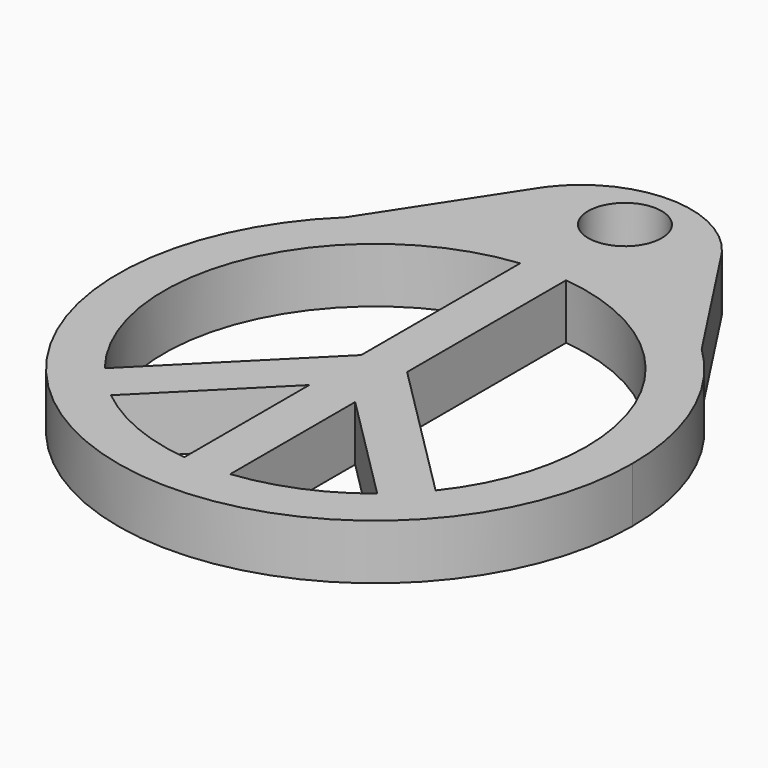
from build123d import *

# Parameters (mm, degrees)
F1_R     = 2
F2_DEPTH = 3


with BuildPart() as f2:
    # F1 (on Top) → F2 (new body)
    with BuildSketch(Plane.XY):
        with BuildLine():
            ThreePointArc((-9.7114153746, 10.0840672063), (-5.4790594428, -12.8833189676), (14, 0))
            ThreePointArc((14, 0), (12.8833189676, 5.4790594428), (9.7114153746, 10.0840672063))
            ThreePointArc((9.7114153746, 10.0840672063), (7.8963049332, 11.5606387541), (5.8606261419, 12.7142857143))
            ThreePointArc((5.8606261419, 12.7142857143), (0, 14), (-5.8606261419, 12.7142857143))
            ThreePointArc((-5.8606261419, 12.7142857143), (-7.8963049332, 11.5606387541), (-9.7114153746, 10.0840672063))
        make_face()
        with BuildLine():
            ThreePointArc((1.25, 11.4318633652), (8.5622718948, 7.6770762664), (11.5, 0))
            ThreePointArc((11.5, 0), (10.8590955773, -3.7855043577), (9.0078185666, -7.1490701963))
            ThreePointArc((9.0078185666, -7.1490701963), (8.1773610714, -8.0858373659), (7.25, -8.9267855357))
            ThreePointArc((7.25, -8.9267855357), (4.4307283524, -10.6121932826), (1.25, -11.4318633652))
            ThreePointArc((1.25, -11.4318633652), (0, -11.5), (-1.25, -11.4318633652))
            ThreePointArc((-1.25, -11.4318633652), (-4.4307283524, -10.6121932826), (-7.25, -8.9267855357))
            ThreePointArc((-7.25, -8.9267855357), (-8.1773610714, -8.0858373659), (-9.0078185666, -7.1490701963))
            ThreePointArc((-9.0078185666, -7.1490701963), (-10.6121856109, 4.4307467271), (-1.25, 11.4318633652))
            ThreePointArc((-1.25, 11.4318633652), (0, 11.5), (1.25, 11.4318633652))
        make_face(mode=Mode.SUBTRACT)
        with BuildLine():
            ThreePointArc((5.8606261419, 12.7142857143), (7.8963049332, 11.5606387541), (9.7114153746, 10.0840672063))
            Line((9.7114153746, 10.0840672063), (5.1961524227, 17))
            ThreePointArc((5.1961524227, 17), (5.9291588604, 14.9192797226), (5.8606261419, 12.7142857143))
        make_face()
        with BuildLine():
            Line((-5.1961524227, 17), (-9.7114153746, 10.0840672063))
            ThreePointArc((-9.7114153746, 10.0840672063), (-7.8963049332, 11.5606387541), (-5.8606261419, 12.7142857143))
            ThreePointArc((-5.8606261419, 12.7142857143), (-5.9291588604, 14.9192797226), (-5.1961524227, 17))
        make_face()
        with BuildLine():
            ThreePointArc((-5.8606261419, 12.7142857143), (0, 14), (5.8606261419, 12.7142857143))
            ThreePointArc((5.8606261419, 12.7142857143), (5.9291588604, 14.9192797226), (5.1961524227, 17))
            ThreePointArc((5.1961524227, 17), (0, 20), (-5.1961524227, 17))
            ThreePointArc((-5.1961524227, 17), (-5.9291588604, 14.9192797226), (-5.8606261419, 12.7142857143))
        make_face()
        with Locations((0, 17)):
            Circle(F1_R, mode=Mode.SUBTRACT)
        with BuildLine():
            Line((1.25, 0.6087483703), (1.25, 11.4318633652))
            ThreePointArc((1.25, 11.4318633652), (0, 11.5), (-1.25, 11.4318633652))
            Line((-1.25, 11.4318633652), (-1.25, 0.6087483703))
            Line((-1.25, 0.6087483703), (-9.0078185666, -7.1490701963))
            ThreePointArc((-9.0078185666, -7.1490701963), (-8.1773610714, -8.0858373659), (-7.25, -8.9267855357))
            Line((-7.25, -8.9267855357), (-1.25, -2.9267855357))
            Line((-1.25, -2.9267855357), (-1.25, -11.4318633652))
            ThreePointArc((-1.25, -11.4318633652), (0, -11.5), (1.25, -11.4318633652))
            Line((1.25, -11.4318633652), (1.25, -2.9267855357))
            Line((1.25, -2.9267855357), (7.25, -8.9267855357))
            ThreePointArc((7.25, -8.9267855357), (8.1773610714, -8.0858373659), (9.0078185666, -7.1490701963))
            Line((9.0078185666, -7.1490701963), (1.25, 0.6087483703))
        make_face()
    extrude(amount=F2_DEPTH)


solid = f2.part
